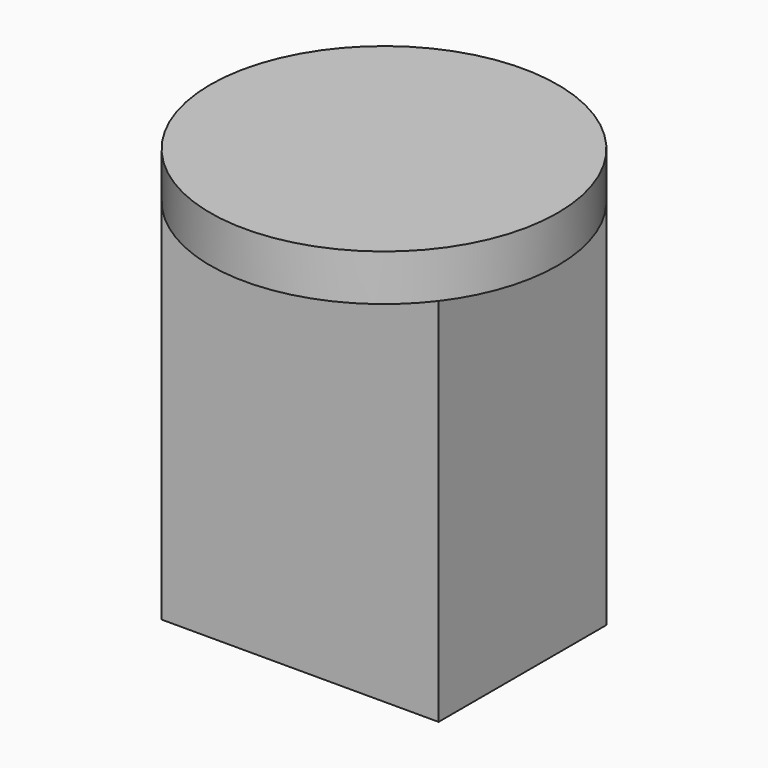
from build123d import *

# Parameters (mm, degrees)
F2_R     = 3.75
F3_DEPTH = 1
F4_W     = 5.9792066569
F4_H     = 4.5275918273
F5_DEPTH = 3
F6_DEPTH = 5


# Not quite as in the source:
# - the program builds the solid bodies; features that only make, move or delete a surface that nothing else refers to are left out


with BuildPart() as f3:
    # F2 (on Top) → F3 (new body)
    with BuildSketch(Plane.XY):
        Circle(F2_R)
    extrude(amount=F3_DEPTH)

    # F4 (on face) → F5 (join)
    with BuildSketch(Plane(origin=(0, 0, 0), x_dir=(1, 0, 0), z_dir=(0, 0, -1))):
        Rectangle(F4_W, F4_H)
    extrude(amount=F5_DEPTH)

    # F6 (add): a face of the model
    f6_faces = [f3.faces().sort_by_distance(p)[0] for p in [
        (0, 0, -3),
    ]]
    extrude(f6_faces, amount=F6_DEPTH)


solid = f3.part
